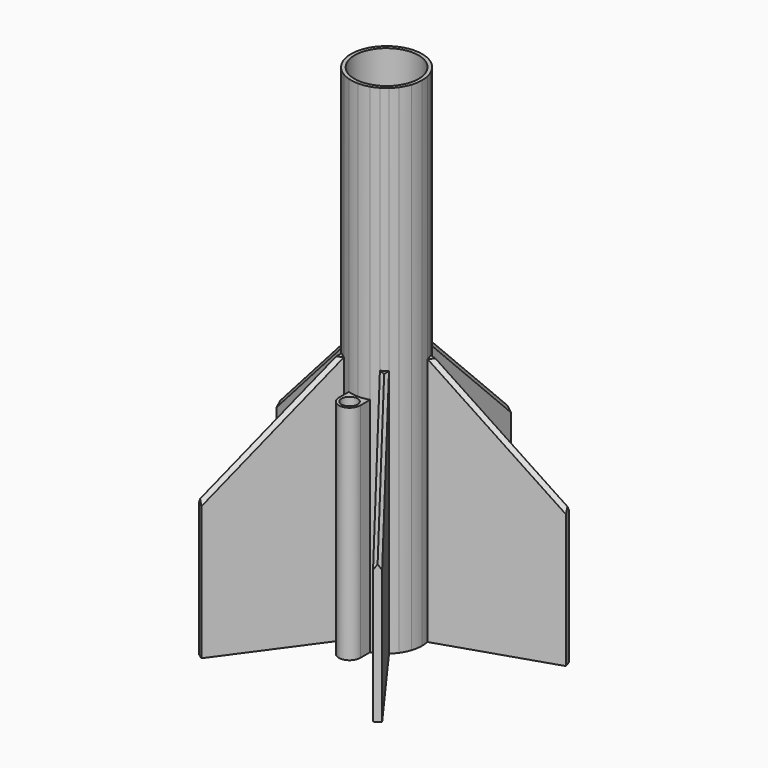
from build123d import *

# Parameters (mm, degrees)
F0_R     = 9
F1_DEPTH = 140
F2_DEPTH = 70
F3_SIZE  = 31
F4_SIZE  = 0.99999
F5_COUNT = 5
F0_R_2   = 2.25
F6_DEPTH = 62.5
F7_START = 63
F0_R_3   = 7.5
F7_DEPTH = 2


# Not quite as in the source:
# - a fillet or chamfer is up to 0.001 mm smaller than in the source, because OpenCascade refuses the exact size


with BuildPart() as f1:
    # F0 (on Top) → F1 (new body)
    with BuildSketch(Plane.XY):
        with BuildLine():
            ThreePointArc((3, -9.5393920142), (8.0622577483, -5.9160797831), (10, 0))
            ThreePointArc((10, 0), (7.4161984871, 6.7082039325), (1, 9.9498743711))
            ThreePointArc((1, 9.9498743711), (0, 10), (-1, 9.9498743711))
            ThreePointArc((-1, 9.9498743711), (-9.9477573381, 1.0208447195), (-3, -9.5393920142))
            ThreePointArc((-3, -9.5393920142), (-1.5175770051, -9.8841772563), (-2.49e-08, -10))
            ThreePointArc((-2.49e-08, -10), (1.5175769805, -9.8841772601), (3, -9.5393920142))
        make_face()
        Circle(F0_R, mode=Mode.SUBTRACT)
    extrude(amount=F1_DEPTH)

    # F0 (on Top) → F2 (join)
    with BuildSketch(Plane.XY):
        with BuildLine():
            ThreePointArc((-1, 9.9498743711), (0, 10), (1, 9.9498743711))
            Line((1, 9.9498743711), (1, 42.4498743711))
            Line((1, 42.4498743711), (-1, 42.4498743711))
            Line((-1, 42.4498743711), (-1, 9.9498743711))
        make_face()
    extrude(amount=F2_DEPTH)

    # F3
    f3_edges = [f1.edges().sort_by_distance(p)[0] for p in [
        (0, 42.449874, 70),
    ]]
    chamfer(f3_edges, length=F3_SIZE)

    # F4 (size 1 in the source; OpenCascade refuses exactly that, so slightly less here)
    f4_edges = [f1.edges().sort_by_distance(p)[0] for p in [
        (-1, 26.949874, 54.5),
        (1, 26.949874, 54.5),
    ]]
    chamfer(f4_edges, length=F4_SIZE)

    # F5: F1 ×5 about axis
    f5_axis = Axis((0, 0, 0), (0, 0, -1))


with BuildPart() as f1_1:
    add(f1.part)
    for i in range(1, F5_COUNT):
        add(f1.part.rotate(f5_axis, i * 360 / F5_COUNT))

    # F0 (on Top) → F6 (join)
    with BuildSketch(Plane.XY):
        with BuildLine():
            ThreePointArc((-3, -13), (-2.1213203524, -10.8786796652), (-2.49e-08, -10))
            ThreePointArc((-2.49e-08, -10), (-1.5175770051, -9.8841772563), (-3, -9.5393920142))
            Line((-3, -9.5393920142), (-3, -13))
        make_face()
        with BuildLine():
            Line((3, -13), (3, -9.5393920142))
            ThreePointArc((3, -9.5393920142), (1.5175769805, -9.8841772601), (-2.49e-08, -10))
            ThreePointArc((-2.49e-08, -10), (2.1213203348, -10.8786796476), (3, -13))
        make_face()
        with BuildLine():
            ThreePointArc((3, -13), (2.1213203348, -10.8786796476), (-2.49e-08, -10))
            ThreePointArc((-2.49e-08, -10), (-2.1213203524, -10.8786796652), (-3, -13))
            ThreePointArc((-3, -13), (0, -16), (3, -13))
        make_face()
        with Locations((0, -13)):
            Circle(F0_R_2, mode=Mode.SUBTRACT)
    extrude(amount=F6_DEPTH)

    # F0 (on Top) → F7 (join)
    with BuildSketch(Plane.XY.offset(F7_START)):
        Circle(F0_R)
        Circle(F0_R_3, mode=Mode.SUBTRACT)
    extrude(amount=F7_DEPTH)


solid = f1_1.part
